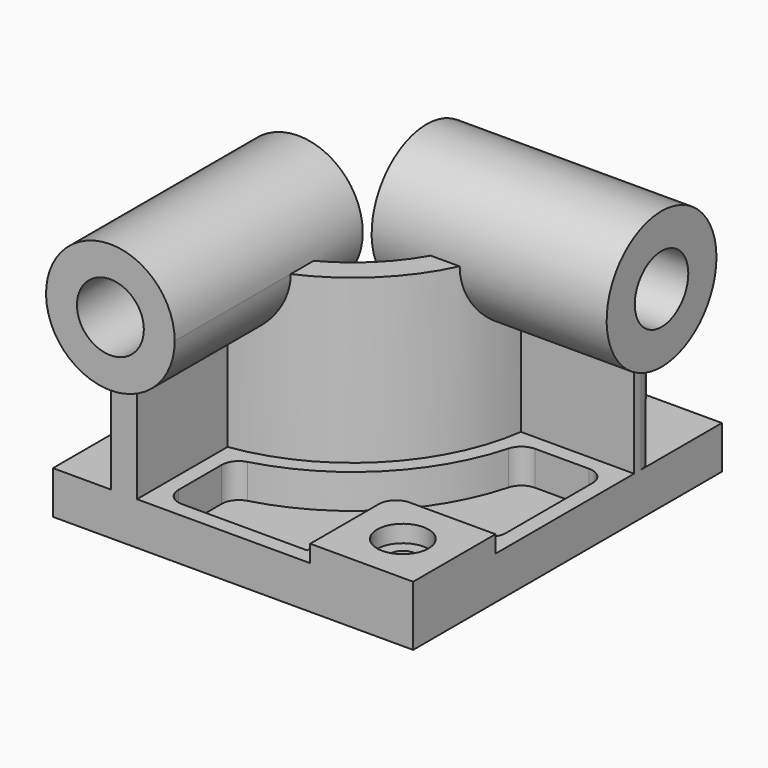
from build123d import *

# Parameters (mm, degrees)
F0_W            = 210
F0_H            = 225
F1_DEPTH        = 25
F3_DEPTH        = 95
F5_DEPTH        = 10
F5_DEPTH_BACK   = 127
F7_DEPTH        = 10
F7_DEPTH_BACK   = 127
F8_W            = 60
F8_H            = 60
F9_DEPTH        = 10
F10_R           = 10
F12_DEPTH       = 20
F14_D           = 15
F14_CBORE_D     = 30
F14_CBORE_DEPTH = 10
F15_T1_DEPTH    = 20
F15_T6_DEPTH    = 80.7094158862
F15_S7_R        = 40
F15_T8_DEPTH    = 42
F15_T12_DEPTH   = 79.5275350517
F15_S13_R       = 40
F15_T14_DEPTH   = 42
F15_T18_DEPTH   = 82.0757730237
F15_S19_R       = 37.5
F15_T20_DEPTH   = 43
F16_R           = 19.5
F17_DEPTH       = 235.001
F18_R           = 19.5
F19_DEPTH       = 220.001


# Not quite as in the source:
# - a fillet or chamfer that OpenCascade refuses, or shapes differently, is made with other operations: its cross-section is extruded or revolved along the edge and cut away or added


with BuildPart() as f1:
    # F0 (on Top) → F1 (new body)
    with BuildSketch(Plane.XY):
        Rectangle(F0_W, F0_H)
    extrude(amount=F1_DEPTH)

    # F2 (on face) → F3 (join)
    with BuildSketch(Plane.XY.offset(25)):
        with BuildLine():
            Line((105, 48.5), (105, 63.5))
            Line((105, 63.5), (25, 63.5))
            ThreePointArc((25, 63.5), (-3.1177490061, -4.3822509939), (-71, -32.5))
            Line((-71, -32.5), (-71, -112.5))
            Line((-71, -112.5), (-56, -112.5))
            Line((-56, -112.5), (-56, -46.4818166789))
            ThreePointArc((-56, -46.4818166789), (7.4888527117, -14.9888527117), (38.9818166789, 48.5))
            Line((38.9818166789, 48.5), (105, 48.5))
        make_face()
    extrude(amount=F3_DEPTH)

    # F4 (on face) → F5 (join, two sides)
    with BuildSketch(Plane.XZ.offset(112.5)) as f5_sk:
        with BuildLine():
            ThreePointArc((-56, 83.2576538583), (-34.4526249034, 96.2829175487), (-26, 120))
            ThreePointArc((-26, 120), (-87.2170824513, 149.0473750966), (-71, 83.2576538583))
            Line((-71, 83.2576538583), (-71, 120))
            Line((-71, 120), (-56, 120))
            Line((-56, 120), (-56, 83.2576538583))
        make_face()
        with BuildLine():
            Line((-71, 120), (-71, 83.2576538583))
            ThreePointArc((-71, 83.2576538583), (-63.5, 82.5), (-56, 83.2576538583))
            Line((-56, 83.2576538583), (-56, 120))
            Line((-56, 120), (-71, 120))
        make_face()
    extrude(amount=F5_DEPTH)
    extrude(f5_sk.sketch, amount=-F5_DEPTH_BACK)

    # F6 (on face) → F7 (join, two sides)
    with BuildSketch(Plane.YZ.offset(105)) as f7_sk:
        with BuildLine():
            Line((48.5, 120), (48.5, 80.7094158862))
            ThreePointArc((48.5, 80.7094158862), (56, 80), (63.5, 80.7094158862))
            Line((63.5, 80.7094158862), (63.5, 120))
            Line((63.5, 120), (48.5, 120))
        make_face()
        with BuildLine():
            ThreePointArc((63.5, 80.7094158862), (86.8220700148, 94.504902432), (96, 120))
            ThreePointArc((96, 120), (30.504902432, 150.8220700148), (48.5, 80.7094158862))
            Line((48.5, 80.7094158862), (48.5, 120))
            Line((48.5, 120), (63.5, 120))
            Line((63.5, 120), (63.5, 80.7094158862))
        make_face()
    extrude(amount=F7_DEPTH)
    extrude(f7_sk.sketch, amount=-F7_DEPTH_BACK)

    # F8 (on face) → F9 (join)
    with BuildSketch(Plane.XY.offset(25)):
        with Locations((75, -82.5)):
            Rectangle(F8_W, F8_H)
    extrude(amount=F9_DEPTH)

    # F10
    f10_edges = [f1.edges().sort_by_distance(p)[0] for p in [
        (45, -52.5, 30),
    ]]
    fillet(f10_edges, radius=F10_R)

    # F11 (on face) → F12 (cut)
    with BuildSketch(Plane.XY.offset(25)):
        with BuildLine():
            ThreePointArc((46.5755076536, 39.5), (13.8528137424, -21.3528137424), (-47, -54.0755076536))
            Line((-47, -54.0755076536), (-47, -103.5))
            Line((-47, -103.5), (36, -103.5))
            Line((36, -103.5), (36, -62.5))
            ThreePointArc((36, -62.5), (41.5649711575, -49.0649711575), (55, -43.5))
            Line((55, -43.5), (96, -43.5))
            Line((96, -43.5), (96, 39.5))
            Line((96, 39.5), (46.5755076536, 39.5))
        make_face()
    extrude(amount=-F12_DEPTH, mode=Mode.SUBTRACT)

    # F14 (through all)
    with Locations(Plane.XY.offset(35)):
        with Locations((75, -82.5)):
            CounterBoreHole(F14_D / 2, F14_CBORE_D / 2, F14_CBORE_DEPTH)

    # F15: fillet of radius 10 on 8 edges, made by hand

    # F15_s2 → F15_t1 (join)
    with BuildSketch(Plane.XY.offset(5)):
        with BuildLine():
            ThreePointArc((-39.6153846154, -52.3231665823), (-44.9420981533, -55.8986609284), (-47, -61.9750971309))
            Line((-47, -61.9750971309), (-47, -54.0755076536))
            ThreePointArc((-47, -54.0755076536), (-43.2938349797, -53.257733876), (-39.6153846154, -52.3231665823))
        make_face()
        with BuildLine():
            ThreePointArc((44.8231665823, 32.1153846154), (48.3986609284, 37.4420981533), (54.4750971309, 39.5))
            Line((54.4750971309, 39.5), (46.5755076536, 39.5))
            ThreePointArc((46.5755076536, 39.5), (45.757733876, 35.7938349797), (44.8231665823, 32.1153846154))
        make_face()
        with BuildLine():
            ThreePointArc((96, 29.5), (93.0710678119, 36.5710678119), (86, 39.5))
            Line((86, 39.5), (96, 39.5))
            Line((96, 39.5), (96, 29.5))
        make_face()
        with BuildLine():
            ThreePointArc((86, -43.5), (93.0710678119, -40.5710678119), (96, -33.5))
            Line((96, -33.5), (96, -43.5))
            Line((96, -43.5), (86, -43.5))
        make_face()
        with BuildLine():
            ThreePointArc((-47, -93.5), (-44.0710678119, -100.5710678119), (-37, -103.5))
            Line((-37, -103.5), (-47, -103.5))
            Line((-47, -103.5), (-47, -93.5))
        make_face()
    extrude(amount=F15_T1_DEPTH)


with BuildPart() as f15_tool4:
    # F15_s5 → F15_t6 (new body)
    with BuildSketch(Plane.XY.offset(25)):
        with BuildLine():
            ThreePointArc((105, 53.5), (102.0710678119, 60.5710678119), (95, 63.5))
            Line((95, 63.5), (105, 63.5))
            Line((105, 63.5), (105, 53.5))
        make_face()
    extrude(amount=F15_T6_DEPTH)

    # F15_s7 → F15_t8 (cut, symmetric)
    with BuildSketch(Plane.YZ.offset(100)):
        with Locations((56, 120)):
            Circle(F15_S7_R)
    extrude(amount=F15_T8_DEPTH, both=True, mode=Mode.SUBTRACT)


with BuildPart() as f1_1:
    add(f1.part)

    # F15_t3: cut F15_tool4
    add(f15_tool4.part, mode=Mode.SUBTRACT)


with BuildPart() as f15_tool10:
    # F15_s11 → F15_t12 (new body)
    with BuildSketch(Plane.XY.offset(25)):
        with BuildLine():
            ThreePointArc((34.5272476662, 63.5), (27.7979818171, 60.8970927486), (24.571846943, 54.4433962264))
            ThreePointArc((24.571846943, 54.4433962264), (24.8929019962, 58.9666406785), (25, 63.5))
            Line((25, 63.5), (34.5272476662, 63.5))
        make_face()
    extrude(amount=F15_T12_DEPTH)

    # F15_s13 → F15_t14 (cut, symmetric)
    with BuildSketch(Plane.YZ.offset(29.5)):
        with Locations((56, 120)):
            Circle(F15_S13_R)
    extrude(amount=F15_T14_DEPTH, both=True, mode=Mode.SUBTRACT)


with BuildPart() as f1_2:
    add(f1_1.part)

    # F15_t9: cut F15_tool10
    add(f15_tool10.part, mode=Mode.SUBTRACT)


with BuildPart() as f15_tool16:
    # F15_s17 → F15_t18 (new body)
    with BuildSketch(Plane.XY.offset(25)):
        with BuildLine():
            ThreePointArc((-71, -42.0272476662), (-68.3970927486, -35.2979818171), (-61.9433962264, -32.071846943))
            ThreePointArc((-61.9433962264, -32.071846943), (-66.4666406785, -32.3929019962), (-71, -32.5))
            Line((-71, -32.5), (-71, -42.0272476662))
        make_face()
    extrude(amount=F15_T18_DEPTH)

    # F15_s19 → F15_t20 (cut, symmetric)
    with BuildSketch(Plane.XZ.offset(37)):
        with Locations((-63.5, 120)):
            Circle(F15_S19_R)
    extrude(amount=F15_T20_DEPTH, both=True, mode=Mode.SUBTRACT)


with BuildPart() as f1_3:
    add(f1_2.part)

    # F15_t15: cut F15_tool16
    add(f15_tool16.part, mode=Mode.SUBTRACT)

    # F16 (on face) → F17 (cut, through all)
    with BuildSketch(Plane.XZ.offset(122.5)):
        with Locations((-63.5, 120)):
            Circle(F16_R)
    extrude(amount=-F17_DEPTH, mode=Mode.SUBTRACT)

    # F18 (on face) → F19 (cut, through all)
    with BuildSketch(Plane.YZ.offset(115)):
        with Locations((56, 120)):
            Circle(F18_R)
    extrude(amount=-F19_DEPTH, mode=Mode.SUBTRACT)


solid = f1_3.part
